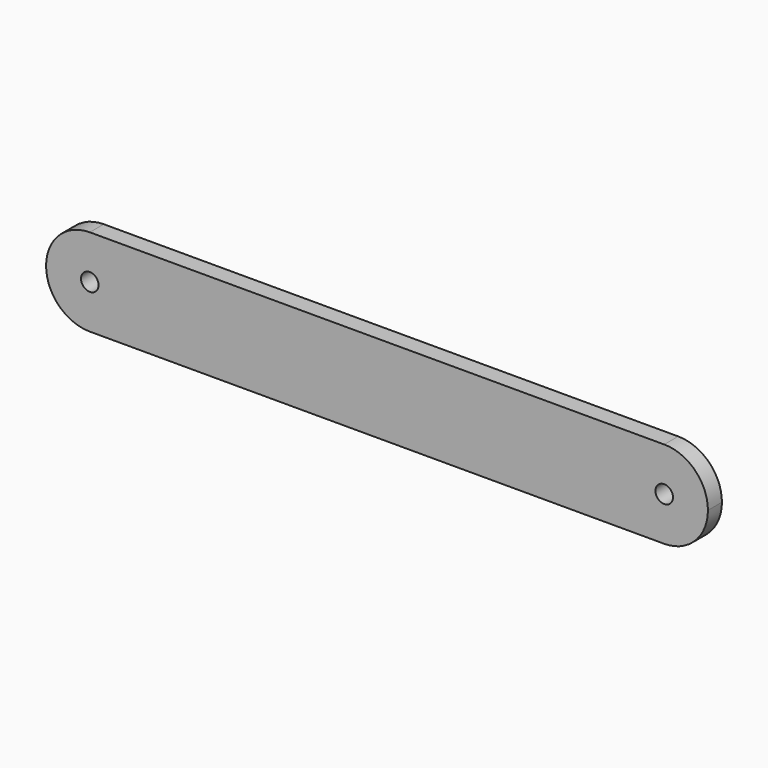
from build123d import *

# Parameters (mm, degrees)
F0_W     = 75.7
F0_H     = 10
F0_R     = 1
F1_DEPTH = 2
F2_R     = 5
F3_R     = 4.99999
F4_R     = 5
F5_R     = 4.99999


# Not quite as in the source:
# - a fillet or chamfer is up to 0.001 mm smaller than in the source, because OpenCascade refuses the exact size


with BuildPart() as f1:
    # F0 (on Front) → F1 (new body)
    with BuildSketch(Plane.XZ):
        with Locations((37.85, -5)):
            Rectangle(F0_W, F0_H)
        with Locations((5, -5)):
            Circle(F0_R, mode=Mode.SUBTRACT)
        with Locations((70.7, -5)):
            Circle(F0_R, mode=Mode.SUBTRACT)
    extrude(amount=F1_DEPTH)

    # F2
    f2_edges = [f1.edges().sort_by_distance(p)[0] for p in [
        (0, -1, 0),
    ]]
    fillet(f2_edges, radius=F2_R)

    # F3 (radius 5 in the source; OpenCascade refuses exactly that, so slightly less here)
    f3_edges = [f1.edges().sort_by_distance(p)[0] for p in [
        (0, -1, -10),
    ]]
    fillet(f3_edges, radius=F3_R)

    # F4
    f4_edges = [f1.edges().sort_by_distance(p)[0] for p in [
        (75.7, -1, -10),
    ]]
    fillet(f4_edges, radius=F4_R)

    # F5 (radius 5 in the source; OpenCascade refuses exactly that, so slightly less here)
    f5_edges = [f1.edges().sort_by_distance(p)[0] for p in [
        (75.7, -1, 0),
    ]]
    fillet(f5_edges, radius=F5_R)


solid = f1.part
